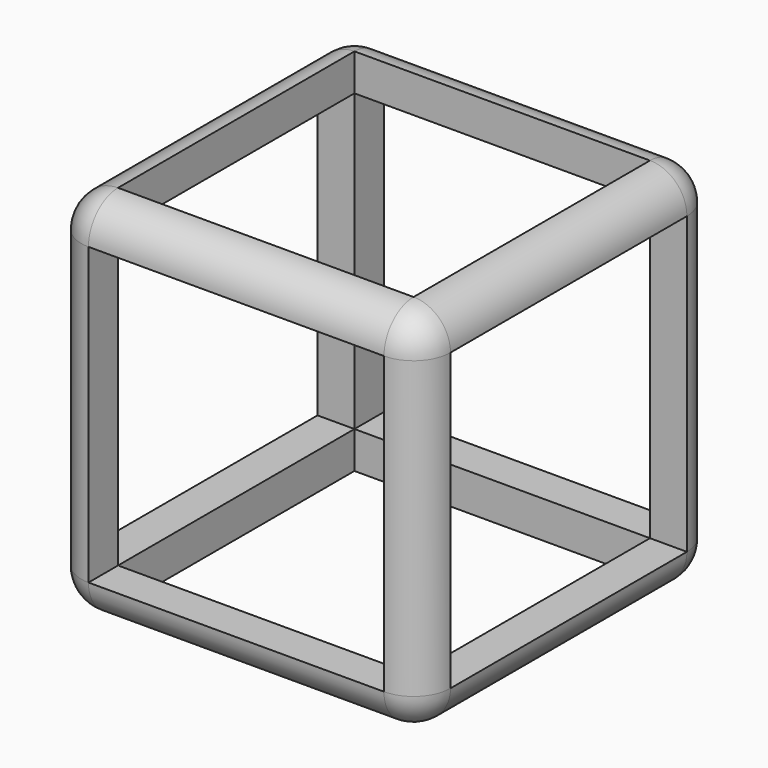
from build123d import *

# Parameters (mm, degrees)
F0_W         = 25.4
F0_H         = 25.4
F1_DEPTH     = 25.4
F2_R         = 2.54
F3_T1_DEPTH  = 20.32
F3_S5_W      = 2.54
F3_S5_H      = 2.54
F3_T6_DEPTH  = 2.54
F3_S11_W     = 2.54
F3_S11_H     = 2.54
F3_T12_DEPTH = 2.54
F4_DEPTH     = 25.401
F5_DEPTH     = 25.401
F6_DEPTH     = 25.401


# Not quite as in the source:
# - a fillet or chamfer that OpenCascade refuses, or shapes differently, is made with other operations: its cross-section is extruded or revolved along the edge and cut away or added


with BuildPart() as f1:
    # F0 (on Front) → F1 (new body)
    with BuildSketch(Plane.XZ):
        with Locations((12.7, -12.7)):
            Rectangle(F0_W, F0_H)
    extrude(amount=F1_DEPTH)

    # F2
    f2_edges = [f1.edges().sort_by_distance(p)[0] for p in [
        (0, 0, -12.7),
        (0, -25.4, -12.7),
        (0, -12.7, -25.4),
        (12.7, 0, -25.4),
        (25.4, 0, -12.7),
        (12.7, 0, 0),
        (0, -12.7, 0),
        (25.4, -12.7, 0),
        (25.4, -12.7, -25.4),
        (25.4, -25.4, -12.7),
        (12.7, -25.4, 0),
    ]]
    fillet(f2_edges, radius=F2_R)

    # F3: fillet of radius 2.54 on 1 edges, made by hand

    # F3_s2 → F3_t1 (cut)
    with BuildSketch(Plane.YZ.offset(2.54)):
        with BuildLine():
            ThreePointArc((-25.4, -22.86), (-24.6560512242, -24.6560512242), (-22.86, -25.4))
            Line((-22.86, -25.4), (-25.4, -25.4))
            Line((-25.4, -25.4), (-25.4, -22.86))
        make_face()
    extrude(amount=F3_T1_DEPTH, mode=Mode.SUBTRACT)


with BuildPart() as f3_tool4:
    # F3_s5 → F3_t6 (new body)
    with BuildSketch(Plane.XZ.offset(22.86)):
        with Locations((1.27, -24.13)):
            Rectangle(F3_S5_W, F3_S5_H)
    extrude(amount=F3_T6_DEPTH)

    # F3_s7 → F3_t8 (revolve, cut)
    with BuildSketch(Plane(origin=(2.54, -22.86, -22.86), x_dir=(0.7071067812, 0, 0.7071067812), z_dir=(0.7071067812, 0, -0.7071067812))):
        with BuildLine():
            ThreePointArc((0, -2.54), (2.54, 0), (0, 2.54))
            Line((0, 2.54), (0, -2.54))
        make_face()
    revolve(axis=Axis((2.54, -22.86, -22.86), (0, -1, 0)), mode=Mode.SUBTRACT)


with BuildPart() as f1_1:
    add(f1.part)

    # F3_t3: cut F3_tool4
    add(f3_tool4.part, mode=Mode.SUBTRACT)


with BuildPart() as f3_tool10:
    # F3_s11 → F3_t12 (new body)
    with BuildSketch(Plane.XZ.offset(22.86)):
        with Locations((24.13, -24.13)):
            Rectangle(F3_S11_W, F3_S11_H)
    extrude(amount=F3_T12_DEPTH)

    # F3_s13 → F3_t14 (revolve, cut)
    with BuildSketch(Plane(origin=(22.86, -22.86, -22.86), x_dir=(-0.7071067812, 0, 0.7071067812), z_dir=(0.7071067812, 0, 0.7071067812))):
        with BuildLine():
            ThreePointArc((0, -2.54), (2.54, 0), (0, 2.54))
            Line((0, 2.54), (0, -2.54))
        make_face()
    revolve(axis=Axis((22.86, -22.86, -22.86), (0, -1, 0)), mode=Mode.SUBTRACT)


with BuildPart() as f1_2:
    add(f1_1.part)

    # F3_t9: cut F3_tool10
    add(f3_tool10.part, mode=Mode.SUBTRACT)

    # F4 (cut, through all): a face of the model
    f4_faces = [f1_2.faces().sort_by_distance(p)[0] for p in [
        (12.7, -12.7, 0),
    ]]
    extrude(f4_faces, amount=-F4_DEPTH, mode=Mode.SUBTRACT)

    # F5 (cut, through all): a face of the model
    f5_faces = [f1_2.faces().sort_by_distance(p)[0] for p in [
        (25.4, -12.7, -12.7),
    ]]
    extrude(f5_faces, amount=-F5_DEPTH, mode=Mode.SUBTRACT)

    # F6 (cut, through all): a face of the model
    f6_faces = [f1_2.faces().sort_by_distance(p)[0] for p in [
        (12.7, 0, -12.7),
    ]]
    extrude(f6_faces, amount=-F6_DEPTH, mode=Mode.SUBTRACT)


solid = f1_2.part
